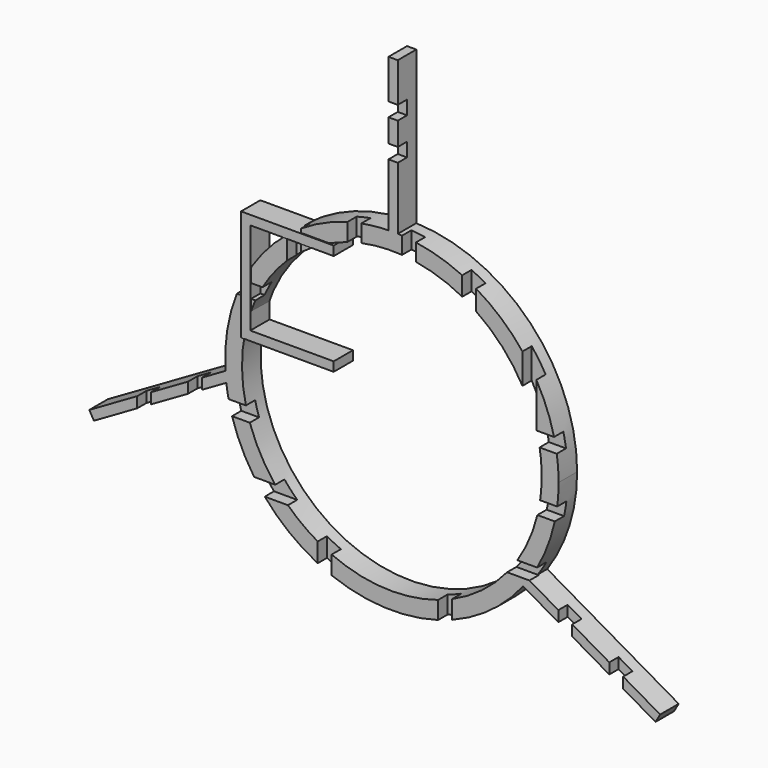
from build123d import *

# Parameters (mm, degrees)
F0_W     = 2
F0_H     = 20
F1_DEPTH = 5.2
F3_R     = 32.3447121386
F4_DEPTH = 5
F5_W     = 13.572675172
F5_H     = 3
F5_W_2   = 3
F5_H_2   = 7.1146996021
F5_W_3   = 2.1339680368
F5_W_4   = 0.2662442029
F5_W_5   = 13.7997193004
F5_W_6   = 30
F5_H_3   = 13.0011811852
F5_H_4   = 30
F5_W_7   = 18.9105942249
F5_H_5   = 10
F5_W_8   = 8
F5_H_6   = 2.1246682657
F5_H_7   = 17.7334510805
F5_W_9   = 0.0894057751
F5_W_10  = 6.9841714074
F5_W_11  = 30.4511226714
F5_H_8   = 23.2589878142
F5_H_9   = 23.0766864568
F5_H_10  = 16.892408269
F5_W_12  = 17.7097696288
F5_W_13  = 22.2877347842
F5_H_11  = 23.447284475
F5_H_12  = 27.4531447118
F5_W_14  = 19.8099045083
F5_W_15  = 9.4498991966
F5_W_16  = 47.1669645049
F6_DEPTH = 2.5


with BuildPart() as f1:
    # F0 (on Front) → F1 (new body)
    with BuildSketch(Plane.XZ):
        Polygon((-32.3928073049, 29.3797243163), (-32.3928073049, 27.3797243163), (-30.3928073049, 27.3797243163), (-12.3928073049, 27.3797243163), (-12.3928073049, 29.3797243163), align=None)
        with Locations((-31.3928073049, 17.3797243163)):
            Rectangle(F0_W, F0_H)
        Polygon((-30.3928073049, 7.3797243163), (-32.3928073049, 7.3797243163), (-32.3928073049, 5.3797243163), (-12.3928073049, 5.3797243163), (-12.3928073049, 7.3797243163), align=None)
    extrude(amount=F1_DEPTH)


with BuildPart() as f4:
    # F3 (on face) → F4 (new body)
    with BuildSketch(Plane.XZ):
        with BuildLine():
            Line((-0.718275291, 68.9771758448), (-0.718275291, 35.9928337396))
            ThreePointArc((-0.718275291, 35.9928337396), (0.2818334687, 35.9988967872), (1.281724709, 35.9771758448))
            Line((1.281724709, 35.9771758448), (1.281724709, 68.9771758448))
            Line((1.281724709, 68.9771758448), (-0.718275291, 68.9771758448))
        make_face()
        with BuildLine():
            ThreePointArc((1.281724709, 35.9771758448), (0.2818334687, 35.9988967872), (-0.718275291, 35.9928337396))
            ThreePointArc((-0.718275291, 35.9928337396), (-26.4593304957, 24.4111415079), (-35.9340729634, -2.1777052736))
            ThreePointArc((-35.9340729634, -2.1777052736), (-35.8506255781, -3.2760716812), (-35.7336132594, -4.3713708863))
            ThreePointArc((-35.7336132594, -4.3713708863), (-9.6415771636, -34.6848668701), (28.3514265226, -22.185504595))
            ThreePointArc((28.3514265226, -22.185504595), (28.9605266738, -21.3842908411), (29.5469914366, -20.5663632431))
            ThreePointArc((29.5469914366, -20.5663632431), (34.3488842011, -10.7774836646), (36, 0))
            ThreePointArc((36, 0), (25.905038984, 24.9985790644), (1.281724709, 35.9771758448))
        make_face()
        Circle(F3_R, mode=Mode.SUBTRACT)
        with BuildLine():
            ThreePointArc((-35.7336132594, -4.3713708863), (-35.8506255781, -3.2760716812), (-35.9340729634, -2.1777052736))
            Line((-35.9340729634, -2.1777052736), (-65.3124515843, -19.1393200788))
            Line((-65.3124515843, -19.1393200788), (-64.3124515843, -20.8713708863))
            Line((-64.3124515843, -20.8713708863), (-35.7336132594, -4.3713708863))
        make_face()
        with BuildLine():
            Line((57.9302648475, -36.9534537874), (29.5469914366, -20.5663632431))
            ThreePointArc((29.5469914366, -20.5663632431), (28.9605266738, -21.3842908411), (28.3514265226, -22.185504595))
            Line((28.3514265226, -22.185504595), (56.9302648475, -38.685504595))
            Line((56.9302648475, -38.685504595), (57.9302648475, -36.9534537874))
        make_face()
    extrude(amount=F4_DEPTH)

    # F5 (on face) → F6 (cut)
    with BuildSketch(Plane.XZ.offset(5)):
        with Locations((-50.7524073439, 4.1931017637)):
            Rectangle(F5_W, F5_H)
        with Locations((-42.4660697579, 9.2504515648)):
            Rectangle(F5_W_2, F5_H_2)
        with Locations((-42.4660697579, 4.1931017637)):
            Rectangle(F5_W_2, F5_H)
        with Locations((-39.8990857395, 4.1931017637)):
            Rectangle(F5_W_3, F5_H)
        Polygon((-40.9660697579, 2.6931017637), (-43.9660697579, 2.6931017637), (-43.9660697579, -10.9778223559), (-40.9660697579, -10.9778223559), (-40.9660697579, -10.3068982363), (-41.2323139608, -10.3068982363), (-41.2323139608, -7.3068982363), (-40.9660697579, -7.3068982363), align=None)
        with Locations((-41.0991918594, -8.8068982363)):
            Rectangle(F5_W_4, F5_H)
        with Locations((-34.0662101077, -8.8068982363)):
            Rectangle(F5_W_5, F5_H)
        with Locations((-21.7747657001, -21.8068982363)):
            Rectangle(F5_W_6, F5_H)
        with Locations((-14.5, -34.2673957348)):
            Rectangle(F5_W_2, F5_H_3)
        with Locations((11.5, -25.582254529)):
            Rectangle(F5_W_2, F5_H_4)
        with Locations((26.4907963276, -19.1589427693)):
            Rectangle(F5_W_7, F5_H)
        with Locations((37.4460934401, -12.6589427693)):
            Rectangle(F5_W_2, F5_H_5)
        with Locations((37.4460934401, -19.1589427693)):
            Rectangle(F5_W_2, F5_H)
        with Locations((42.9460934401, -19.1589427693)):
            Rectangle(F5_W_8, F5_H)
        with Locations((37.4460934401, -6.5966086365)):
            Rectangle(F5_W_2, F5_H_6)
        Polygon((21.3408830383, -7.6589427693), (35.9460934401, -7.6589427693), (35.9460934401, -5.5342745036), (38.9460934401, -5.5342745036), (38.9460934401, -7.6589427693), (46.9460934401, -7.6589427693), (46.9460934401, -4.6589427693), (21.3408830383, -4.6589427693), align=None)
        with Locations((37.4460934401, -29.5256683096)):
            Rectangle(F5_W_2, F5_H_7)
        Polygon((46.9460934401, -7.6589427693), (46.9460934401, -17.6589427693), (47.0354992151, -17.6589427693), (47.0354992151, -20.6589427693), (46.9460934401, -20.6589427693), (46.9460934401, -41.1515384912), (49.9460934401, -41.1515384912), (49.9460934401, -7.6589427693), align=None)
        with Locations((46.9907963276, -19.1589427693)):
            Rectangle(F5_W_9, F5_H)
        with Locations((48.4460934401, -6.1589427693)):
            Rectangle(F5_W_2, F5_H)
        with Locations((53.4381791438, -6.1589427693)):
            Rectangle(F5_W_10, F5_H)
        with Locations((39.7508572787, 6.8410572307)):
            Rectangle(F5_W_11, F5_H)
        with Locations((-8.0932132453, 35.8674060553)):
            Rectangle(F5_W_2, F5_H_8)
        with Locations((3.7013028025, 37.945441626)):
            Rectangle(F5_W_2, F5_H_9)
        with Locations((-53.4660697579, -9.5130702171)):
            Rectangle(F5_W_2, F5_H_10)
        with Locations((-27.079188149, -68.7113851728)):
            Rectangle(F5_W_12, F5_H)
        with Locations((-2.4145045318, 58.9837848544)):
            Rectangle(F5_W_13, F5_H)
        Polygon((-19.5932132453, 38.1955653429), (-22.5932132453, 38.1955653429), (-22.5932132453, 0.1370755699), (-22.5932132453, -8.6032444029), (-19.5932132453, -8.6032444029), align=None)
        with Locations((16.7013028025, 29.8444582149)):
            Rectangle(F5_W_2, F5_H_11)
        with Locations((29.7013028025, 22.2506034889)):
            Rectangle(F5_W_2, F5_H_12)
        with Locations((2.0907674916, 50.9850047922)):
            Rectangle(F5_W_14, F5_H)
        with Locations((-32.0334173739, 14.8294658735)):
            Rectangle(F5_W_15, F5_H)
        with Locations((18.230658723, -57.7113851728)):
            Rectangle(F5_W_16, F5_H)
    extrude(amount=-F6_DEPTH, mode=Mode.SUBTRACT)


solid = Compound([f1.part, f4.part])
